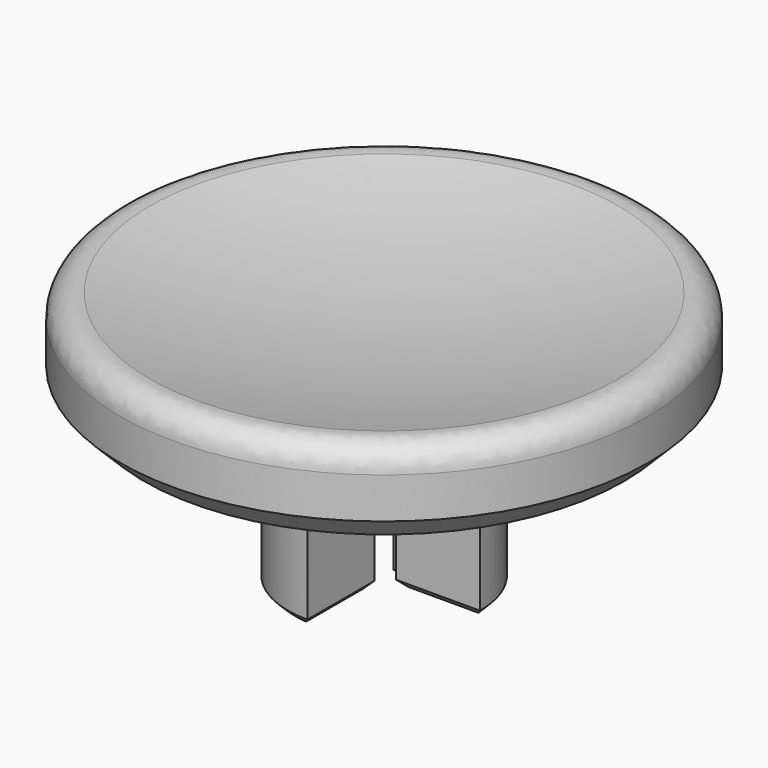
from build123d import *

# Parameters (mm, degrees)
F0_W     = 5.5
F0_H     = 0.5
F2_SIZE  = 1
F3_R     = 1
F5_DEPTH = 6.5
F6_SIZE  = 0.3


with BuildPart() as f1:
    # F0 (on Front) → F1 (revolve)
    with BuildSketch(Plane.XZ):
        with BuildLine():
            ThreePointArc((11, 4), (5.5509008278, 2.8767272628), (0, 2.5))
            Line((0, 2.5), (0, 0))
            Line((0, 0), (5.5, 0))
            Line((5.5, 0), (11, 0))
            Line((11, 0), (11, 4))
        make_face()
        with Locations((2.75, -0.25)):
            Rectangle(F0_W, F0_H)
    revolve(axis=Axis((0, 0, 1.25), (0, 0, -1)))

    # F2
    f2_edges = [f1.edges().sort_by_distance(p)[0] for p in [
        (-11, 0, 0),
    ]]
    chamfer(f2_edges, length=F2_SIZE)

    # F3
    f3_edges = [f1.edges().sort_by_distance(p)[0] for p in [
        (-11, 0, 4),
    ]]
    fillet(f3_edges, radius=F3_R)

    # F4 (on face) → F5 (join)
    with BuildSketch(Plane(origin=(0, 0, -0.5), x_dir=(1, 0, 0), z_dir=(0, 0, -1))):
        with BuildLine():
            ThreePointArc((-0.5, 0), (-0.3535533906, 0.3535533906), (0, 0.5))
            Line((0, 0.5), (0, 4))
            ThreePointArc((0, 4), (-2.8284271247, 2.8284271247), (-4, 0))
            Line((-4, 0), (-0.5, 0))
        make_face()
        with BuildLine():
            Line((4, 0), (0.5, 0))
            ThreePointArc((0.5, 0), (0.3535533906, -0.3535533906), (0, -0.5))
            Line((0, -0.5), (0, -4))
            ThreePointArc((0, -4), (2.8284271247, -2.8284271247), (4, 0))
        make_face()
    extrude(amount=F5_DEPTH)

    # F6
    f6_edges = [f1.edges().sort_by_distance(p)[0] for p in [
        (0, -2.25, -7),
        (-2.828427, -2.828427, -7),
        (-2.25, 0, -7),
        (-0.353553, -0.353553, -7),
        (0.353553, 0.353553, -7),
        (2.25, 0, -7),
        (2.828427, 2.828427, -7),
        (0, 2.25, -7),
    ]]
    chamfer(f6_edges, length=F6_SIZE)


solid = f1.part
